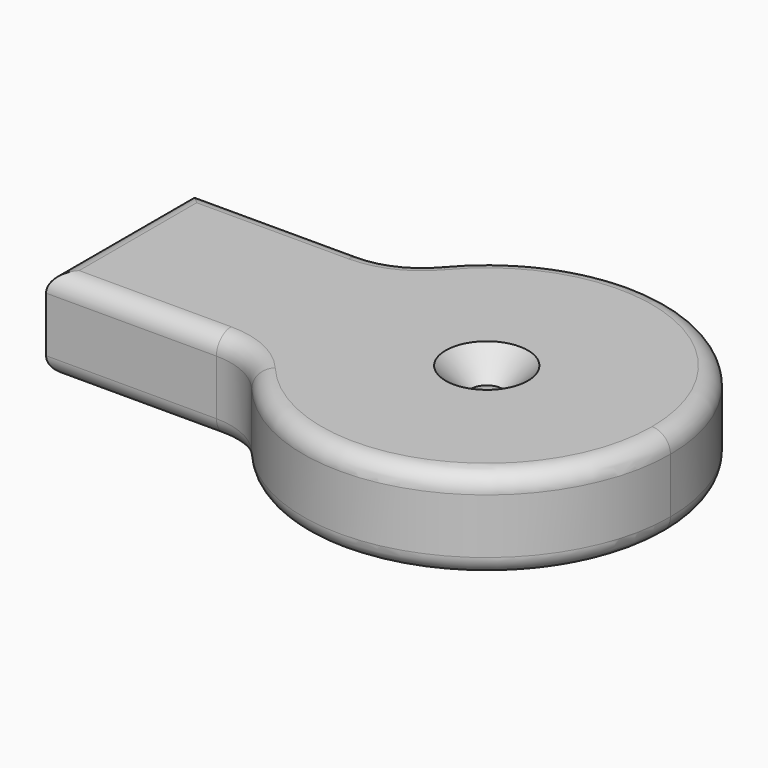
from build123d import *

# Parameters (mm, degrees)
F1_DEPTH       = 12.5
F2_R           = 20
F3_R           = 5
F5_D           = 8.5
F5_CSINK_D     = 22.4
F5_CSINK_ANGLE = 90


with BuildPart() as f1:
    # F0 (on Top) → F1 (new body, symmetric)
    with BuildSketch(Plane.XY):
        with BuildLine():
            ThreePointArc((-43.30127, -25), (-50, 0), (-43.30127, 25))
            Line((-43.30127, 25), (-100, 25))
            Line((-100, 25), (-100, -25))
            Line((-100, -25), (-43.30127, -25))
        make_face()
        with BuildLine():
            ThreePointArc((-43.30127, -25), (12.940952, -48.296291), (50, 0))
            ThreePointArc((50, 0), (12.940952, 48.296291), (-43.30127, 25))
            ThreePointArc((-43.30127, 25), (-50, 0), (-43.30127, -25))
        make_face()
    extrude(amount=F1_DEPTH, both=True)

    # F2
    f2_edges = [f1.edges().sort_by_distance(p)[0] for p in [
        (-43.30127, -25, 0),
        (-43.30127, 25, 0),
    ]]
    fillet(f2_edges, radius=F2_R)

    # F3
    f3_edges = [f1.edges().sort_by_distance(p)[0] for p in [
        (-76.809513, -25, 12.5),
        (-45.167484, -26.873461, 12.5),
        (-100, 0, 12.5),
        (50, 0, 12.5),
        (-76.809513, 25, 12.5),
        (-45.167484, 26.873461, 12.5),
        (-76.809513, -25, -12.5),
        (-45.167484, -26.873461, -12.5),
        (-100, 0, -12.5),
        (50, 0, -12.5),
        (-76.809513, 25, -12.5),
        (-45.167484, 26.873461, -12.5),
    ]]
    fillet(f3_edges, radius=F3_R)

    # F5 (through all)
    with Locations(Plane.XY.offset(12.5)):
        with Locations((0, 0)):
            CounterSinkHole(F5_D / 2, F5_CSINK_D / 2, counter_sink_angle=F5_CSINK_ANGLE)


solid = f1.part
